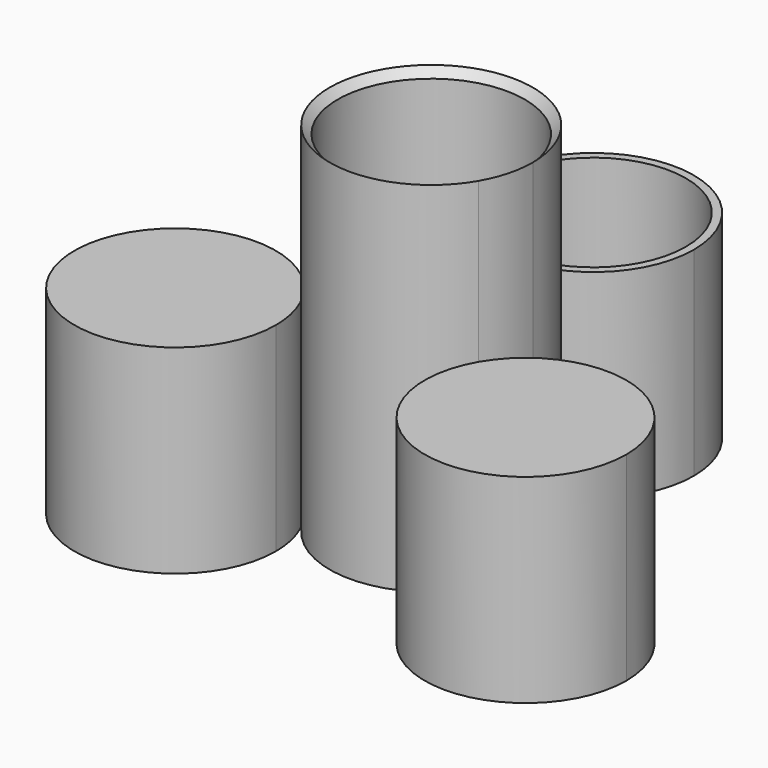
from build123d import *

# Parameters (mm, degrees)
F0_R     = 11.75
F1_DEPTH = 45
F2_DEPTH = 25
F3_SIZE  = 0.99999
F4_R     = 11.65
F5_DEPTH = 23


# Not quite as in the source:
# - a fillet or chamfer is up to 0.001 mm smaller than in the source, because OpenCascade refuses the exact size
# - a feature names something its author has since deleted; it is built from what else it names


with BuildPart() as f1:
    # F0 (on Top) → F1 (new body)
    with BuildSketch(Plane.XY):
        with BuildLine():
            ThreePointArc((11.0418237302, -6.3750002911), (12.3155542417, -3.2999429874), (12.75, 0))
            ThreePointArc((12.75, 0), (9.0156114816, 9.0156114386), (6.08e-08, 12.75))
            ThreePointArc((6.08e-08, 12.75), (-11.0418238613, 6.375000064), (-11.0418239417, -6.3749999247))
            ThreePointArc((-11.0418239417, -6.3749999247), (-2.116e-07, -12.75), (11.0418237302, -6.3750002911))
        make_face()
        Circle(F0_R, mode=Mode.SUBTRACT)
    extrude(amount=F1_DEPTH)

    # F0 (on Top) → F2 (join)
    with BuildSketch(Plane.XY):
        with BuildLine():
            ThreePointArc((11.0418237302, -6.3750002911), (12.3155542417, -3.2999429874), (12.75, 0))
            ThreePointArc((12.75, 0), (9.0156114816, 9.0156114386), (6.08e-08, 12.75))
            ThreePointArc((6.08e-08, 12.75), (-11.0418238613, 6.375000064), (-11.0418239417, -6.3749999247))
            ThreePointArc((-11.0418239417, -6.3749999247), (-2.116e-07, -12.75), (11.0418237302, -6.3750002911))
        make_face()
        Circle(F0_R, mode=Mode.SUBTRACT)
    extrude(amount=F2_DEPTH)

    # F3 (size 1 in the source; OpenCascade refuses exactly that, so slightly less here)
    f3_edges = [f1.edges().sort_by_distance(p)[0] for p in [
        (-11.75, 0, 45),
    ]]
    chamfer(f3_edges, length=F3_SIZE)


with BuildPart() as f2:
    # F0 (on Top) → F2, piece 2 (new body)
    with BuildSketch(Plane.XY):
        with BuildLine():
            ThreePointArc((34.6470452561, -12.7), (25.2711060143, -0.4810382539), (11.0418237302, -6.3750002911))
            ThreePointArc((11.0418237302, -6.3750002911), (18.7229844979, -24.9189617461), (34.6470452561, -12.7))
        make_face()
    extrude(amount=F2_DEPTH)


with BuildPart() as f2b:
    # F0 (on Top) → F2, piece 3 (new body)
    with BuildSketch(Plane.XY):
        with BuildLine():
            ThreePointArc((-9.3470452561, -12.7), (-9.7780835648, -9.4259390375), (-11.0418239417, -6.3749999247))
            ThreePointArc((-11.0418239417, -6.3749999247), (-34.2160069474, -15.9740609625), (-9.3470452561, -12.7))
        make_face()
    extrude(amount=F2_DEPTH)


with BuildPart() as f2c:
    # F0 (on Top) → F2, piece 4 (new body)
    with BuildSketch(Plane.XY):
        with BuildLine():
            ThreePointArc((12.65, 25.4), (-8.9449008035, 34.3449007605), (6.08e-08, 12.75))
            ThreePointArc((6.08e-08, 12.75), (8.9449008035, 16.4550992395), (12.65, 25.4))
        make_face()
    extrude(amount=F2_DEPTH)

    # F4 (on face) → F5 (cut)
    with BuildSketch(Plane.XY.offset(25)):
        with Locations((0, 25.4)):
            Circle(F4_R)
    extrude(amount=-F5_DEPTH, mode=Mode.SUBTRACT)


solid = Compound([f1.part, f2.part, f2b.part, f2c.part])
